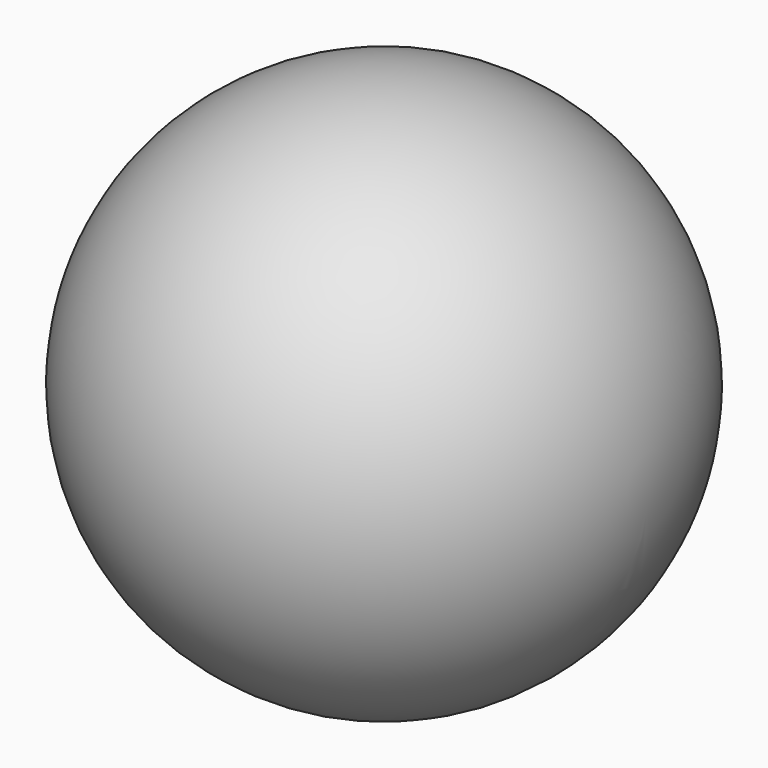
from build123d import *


# Not quite as in the source:
# - the program builds the solid bodies; features that only make, move or delete a surface that nothing else refers to are left out


with BuildPart() as f1:
    # F0 (on Front) → F1 (revolve)
    with BuildSketch(Plane.XZ):
        with BuildLine():
            ThreePointArc((-28.3283509522, 0), (0, -28.3283509522), (28.3283509522, 0))
            Line((28.3283509522, 0), (-28.3283509522, 0))
        make_face()
    revolve(axis=Axis((0, 0, 0), (1, 0, 0)))


solid = f1.part
